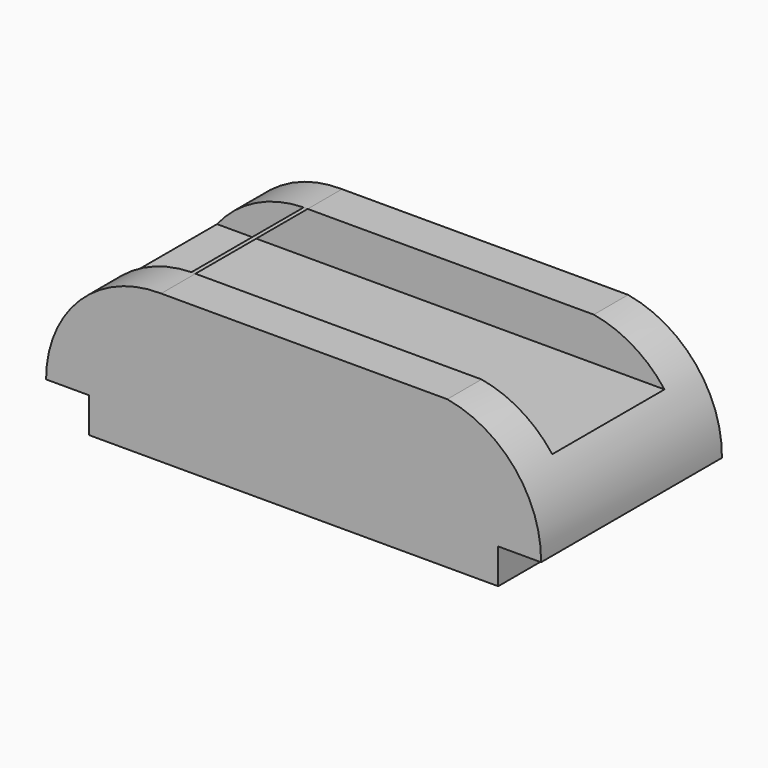
from build123d import *

# Parameters (mm, degrees)
F1_DEPTH      = 29
F2_W          = 36
F2_H          = 11
F3_DEPTH      = 66.5054850399
F3_DEPTH_BACK = 60.4995857167


with BuildPart() as f1:
    # F0 (on Front) → F1 (new body, symmetric)
    with BuildSketch(Plane.XZ):
        with BuildLine():
            Line((-55.504484674, 9), (-55.504484674, 0))
            Line((-55.504484674, 0), (49.495515326, 0))
            Line((49.495515326, 0), (49.495515326, 9))
            Line((49.495515326, 9), (60.495515326, 9))
            ThreePointArc((60.495515326, 9), (53.8144067162, 27.9423579991), (36.4278033617, 38))
            Line((36.4278033617, 38), (-36.987580359, 38))
            ThreePointArc((-36.987580359, 38), (-57.8286498328, 29.6910356314), (-66.504484674, 9))
            Line((-66.504484674, 9), (-55.504484674, 9))
        make_face()
    extrude(amount=F1_DEPTH, both=True)

    # F2 (on Right) → F3 (cut, two sides)
    with BuildSketch(Plane.YZ) as f3_sk:
        with Locations((0, 32.5)):
            Rectangle(F2_W, F2_H)
    extrude(amount=-F3_DEPTH, mode=Mode.SUBTRACT)
    extrude(f3_sk.sketch, amount=F3_DEPTH_BACK, mode=Mode.SUBTRACT)


solid = f1.part
